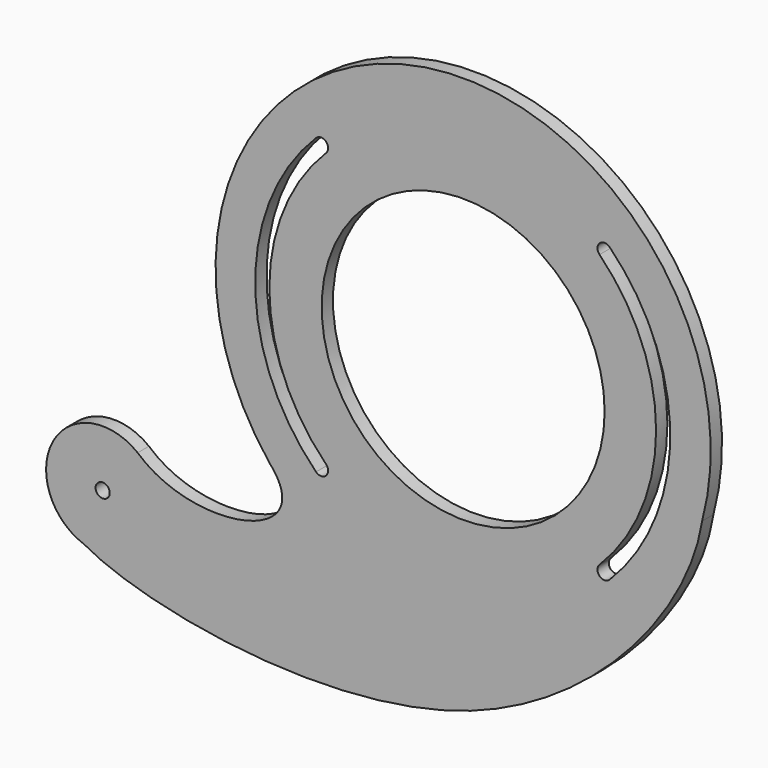
from build123d import *

# Parameters (mm, degrees)
F0_R     = 5
F0_R_2   = 100
F1_DEPTH = 10


# Not quite as in the source:
# - ends of sketch curves that miss each other by under 0.0002 mm in the source are joined


with BuildPart() as f1:
    # F0 (on Front) → F1 (new body)
    with BuildSketch(Plane.XZ):
        with BuildLine():
            add(Edge.make_bspline(
                [(169.1493929479, -45.6158926146), (159.7651292122, -107.4219847214), (22.7183427382, -273.4801182779), (-224.8579575674, -226.7328438), (-267.6564696794, -202.0572125126)],
                knots=[0, 0, 0, 0, 0.4871765071, 1, 1, 1, 1], degree=3))
            ThreePointArc((169.1493929479, -45.6158926146), (-35.404456431, 171.5122555076), (-136.3616027906, -109.1914398753))
            add(Edge.make_bspline(
                [(-229.8119745952, -132.8222825671), (-188.6496121839, -169.4869168537), (-99.4743329729, -150.4504772299), (-136.3616027906, -109.1914398753)],
                knots=[0, 0, 0, 0, 96.391849846, 96.391849846, 96.391849846, 96.391849846], degree=3))
            ThreePointArc((-229.8119745952, -132.8222825671), (-289.6255876831, -145.0881241092), (-267.6564696794, -202.0572125126))
        make_face()
        with Locations((-254.5268251568, -164.2734536378)):
            Circle(F0_R, mode=Mode.SUBTRACT)
        with BuildLine():
            ThreePointArc((-96.6455557461, 97.0129985964), (-136.73540255, 0.1825598604), (-96.6455557461, -96.6478788756))
            ThreePointArc((-96.6455557461, -96.6478788756), (-96.6478779601, -103.7189453909), (-103.7189453903, -103.7166222615))
            ThreePointArc((-103.7189453903, -103.7166222615), (-146.7353999615, 0.1825598604), (-103.7189444749, 104.0817410675))
            ThreePointArc((-103.7189444749, 104.0817410675), (-96.6478779601, 104.0840651118), (-96.6455557461, 97.0129985964))
        make_face(mode=Mode.SUBTRACT)
        with Locations((0.2485292707, 0.1825598604)):
            Circle(F0_R_2, mode=Mode.SUBTRACT)
        with BuildLine():
            ThreePointArc((96.6478838863, -96.2804310179), (136.6228090286, 0.1825598604), (96.6478838863, 96.6455507387))
            ThreePointArc((96.6478838863, 96.6455507387), (96.6455499466, 103.7166173731), (103.7166173736, 103.7189505206))
            ThreePointArc((103.7166173736, 103.7189505206), (146.6228067875, 0.1825598604), (103.7166165815, -103.3538300071))
            ThreePointArc((103.7166165815, -103.3538300071), (96.6455499466, -103.3514976522), (96.6478838863, -96.2804310179))
        make_face(mode=Mode.SUBTRACT)
    extrude(amount=F1_DEPTH)


solid = f1.part
